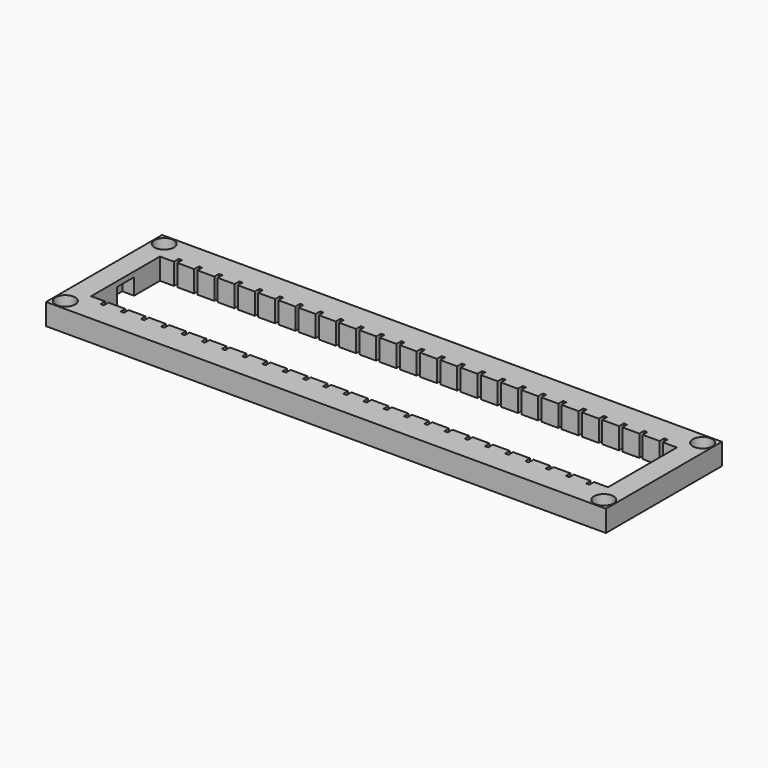
from build123d import *

# Parameters (mm, degrees)
F0_W           = 6.35
F0_H           = 6.35
F1_DEPTH       = 6.35
F2_D           = 3
F2_DEPTH       = 8
F2_CBORE_D     = 5.8
F2_CBORE_DEPTH = 3.5
F2_TIP         = 0.9012909285
F3_W           = 3.5
F3_H           = 6.35
F4_DEPTH       = 4.85


# Not quite as in the source:
# - a feature names something its author has since deleted; it is built from what else it names


with BuildPart() as f1:
    # F0 (on Top) → F1 (new body)
    with BuildSketch(Plane.XY):
        Polygon((-76.65, -21.5), (76.65, -21.5), (76.65, -15.15), (83, -15.15), (83, 15.15), (76.65, 15.15), (76.65, 21.5), (-76.65, 21.5), (-76.65, 15.15), (-83, 15.15), (-83, -15.15), (-76.65, -15.15), align=None)
        Polygon((71.5, 14.5), (72.5, 14.5), (72.5, 12.75), (76.65, 12.75), (76.65, -12.75), (72.5, -12.75), (72.5, -14.5), (71.5, -14.5), (71.5, -12.75), (66.5, -12.75), (66.5, -14.5), (65.5, -14.5), (65.5, -12.75), (60.5, -12.75), (60.5, -14.5), (59.5, -14.5), (59.5, -12.75), (54.5, -12.75), (54.5, -14.5), (53.5, -14.5), (53.5, -12.75), (48.5, -12.75), (48.5, -14.5), (47.5, -14.5), (47.5, -12.75), (42.5, -12.75), (42.5, -14.5), (41.5, -14.5), (41.5, -12.75), (36.5, -12.75), (36.5, -14.5), (35.5, -14.5), (35.5, -12.75), (30.5, -12.75), (30.5, -14.5), (29.5, -14.5), (29.5, -12.75), (24.5, -12.75), (24.5, -14.5), (23.5, -14.5), (23.5, -12.75), (18.5, -12.75), (18.5, -14.5), (17.5, -14.5), (17.5, -12.75), (12.5, -12.75), (12.5, -14.5), (11.5, -14.5), (11.5, -12.75), (6.5, -12.75), (6.5, -14.5), (5.5, -14.5), (5.5, -12.75), (0.5, -12.75), (0.5, -14.5), (-0.5, -14.5), (-0.5, -12.75), (-5.5, -12.75), (-5.5, -14.5), (-6.5, -14.5), (-6.5, -12.75), (-11.5, -12.75), (-11.5, -14.5), (-12.5, -14.5), (-12.5, -12.75), (-17.5, -12.75), (-17.5, -14.5), (-18.5, -14.5), (-18.5, -12.75), (-23.5, -12.75), (-23.5, -14.5), (-24.5, -14.5), (-24.5, -12.75), (-29.5, -12.75), (-29.5, -14.5), (-30.5, -14.5), (-30.5, -12.75), (-35.5, -12.75), (-35.5, -14.5), (-36.5, -14.5), (-36.5, -12.75), (-41.5, -12.75), (-41.5, -14.5), (-42.5, -14.5), (-42.5, -12.75), (-47.5, -12.75), (-47.5, -14.5), (-48.5, -14.5), (-48.5, -12.75), (-53.5, -12.75), (-53.5, -14.5), (-54.5, -14.5), (-54.5, -12.75), (-59.5, -12.75), (-59.5, -14.5), (-60.5, -14.5), (-60.5, -12.75), (-65.5, -12.75), (-65.5, -14.5), (-66.5, -14.5), (-66.5, -12.75), (-71.5, -12.75), (-71.5, -14.5), (-72.5, -14.5), (-72.5, -12.75), (-76.65, -12.75), (-76.65, 12.75), (-72.5, 12.75), (-72.5, 14.5), (-71.5, 14.5), (-71.5, 12.75), (-66.5, 12.75), (-66.5, 14.5), (-65.5, 14.5), (-65.5, 12.75), (-60.5, 12.75), (-60.5, 14.5), (-59.5, 14.5), (-59.5, 12.75), (-54.5, 12.75), (-54.5, 14.5), (-53.5, 14.5), (-53.5, 12.75), (-48.5, 12.75), (-48.5, 14.5), (-47.5, 14.5), (-47.5, 12.75), (-42.5, 12.75), (-42.5, 14.5), (-41.5, 14.5), (-41.5, 12.75), (-36.5, 12.75), (-36.5, 14.5), (-35.5, 14.5), (-35.5, 12.75), (-30.5, 12.75), (-30.5, 14.5), (-29.5, 14.5), (-29.5, 12.75), (-24.5, 12.75), (-24.5, 14.5), (-23.5, 14.5), (-23.5, 12.75), (-18.5, 12.75), (-18.5, 14.5), (-17.5, 14.5), (-17.5, 12.75), (-12.5, 12.75), (-12.5, 14.5), (-11.5, 14.5), (-11.5, 12.75), (-6.5, 12.75), (-6.5, 14.5), (-5.5, 14.5), (-5.5, 12.75), (-0.5, 12.75), (-0.5, 14.5), (0.5, 14.5), (0.5, 12.75), (5.5, 12.75), (5.5, 14.5), (6.5, 14.5), (6.5, 12.75), (11.5, 12.75), (11.5, 14.5), (12.5, 14.5), (12.5, 12.75), (17.5, 12.75), (17.5, 14.5), (18.5, 14.5), (18.5, 12.75), (23.5, 12.75), (23.5, 14.5), (24.5, 14.5), (24.5, 12.75), (29.5, 12.75), (29.5, 14.5), (30.5, 14.5), (30.5, 12.75), (35.5, 12.75), (35.5, 14.5), (36.5, 14.5), (36.5, 12.75), (41.5, 12.75), (41.5, 14.5), (42.5, 14.5), (42.5, 12.75), (47.5, 12.75), (47.5, 14.5), (48.5, 14.5), (48.5, 12.75), (53.5, 12.75), (53.5, 14.5), (54.5, 14.5), (54.5, 12.75), (59.5, 12.75), (59.5, 14.5), (60.5, 14.5), (60.5, 12.75), (65.5, 12.75), (65.5, 14.5), (66.5, 14.5), (66.5, 12.75), (71.5, 12.75), align=None, mode=Mode.SUBTRACT)
        with Locations((-79.825, 18.325)):
            Rectangle(F0_W, F0_H)
        with Locations((-79.825, -18.325)):
            Rectangle(F0_W, F0_H)
        with Locations((79.825, -18.325)):
            Rectangle(F0_W, F0_H)
        with Locations((79.825, 18.325)):
            Rectangle(F0_W, F0_H)
    extrude(amount=-F1_DEPTH)

    # F2
    with Locations(Plane.XY):
        with Locations((-79.825, 18.325), (-79.825, -18.325), (79.825, 18.325), (79.825, -18.325)):
            CounterBoreHole(F2_D / 2, F2_CBORE_D / 2, F2_CBORE_DEPTH, depth=F2_DEPTH)
            with Locations((0, 0, -(F2_DEPTH + F2_TIP / 2))):  # 118° drill point
                Cone(0, F2_D / 2, F2_TIP, mode=Mode.SUBTRACT)

    # F3 (on face) → F4 (cut)
    with BuildSketch(Plane(origin=(0, 0, -6.35), x_dir=(1, 0, 0), z_dir=(0, 0, -1))):
        with Locations((-78.4, 0)):
            Rectangle(F3_W, F3_H)
        with Locations((78.4, 0)):
            Rectangle(F3_W, F3_H)
    extrude(amount=-F4_DEPTH, mode=Mode.SUBTRACT)


solid = f1.part
